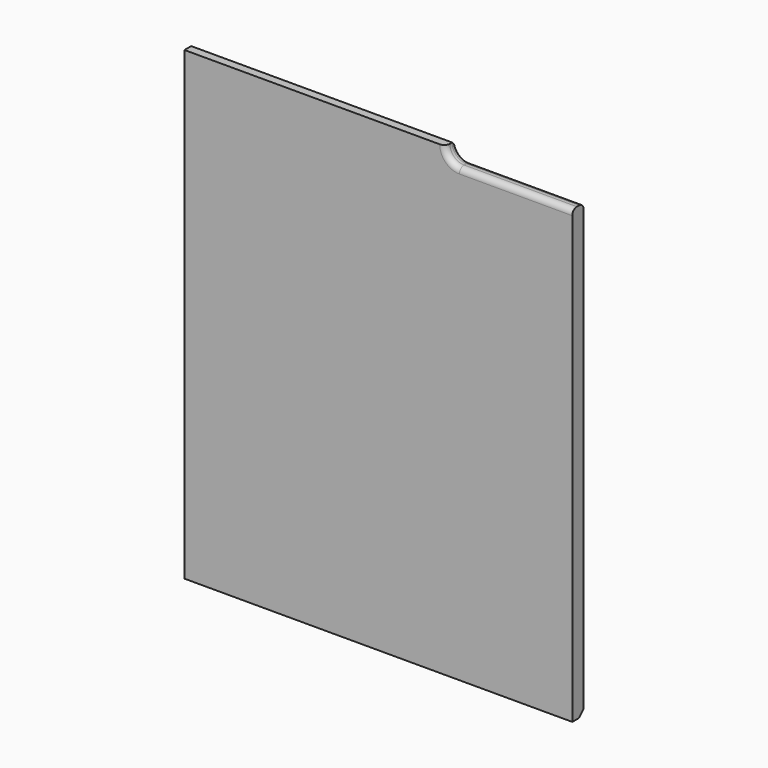
from build123d import *

# Parameters (mm, degrees)
F1_DEPTH    = 12.7
F2_R        = 5.08
F3_T1_DEPTH = 255.9982991577
F3_T3_DEPTH = 445.2282991577
F3_T5_DEPTH = 375.3782991577


# Not quite as in the source:
# - a fillet or chamfer that OpenCascade refuses, or shapes differently, is made with other operations: its cross-section is extruded or revolved along the edge and cut away or added


with BuildPart() as f1:
    # F0 (on Front) → F1 (new body)
    with BuildSketch(Plane.XZ):
        with BuildLine():
            Line((55.5559131622, 244.2450298561), (-179.3940868378, 244.2450298561))
            Line((-179.3940868378, 244.2450298561), (-179.3940868378, -174.8549701439))
            Line((-179.3940868378, -174.8549701439), (169.8559131622, -174.8549701439))
            Line((169.8559131622, -174.8549701439), (169.8559131622, 231.5450298561))
            Line((169.8559131622, 231.5450298561), (68.2559131622, 231.5450298561))
            ThreePointArc((68.2559131622, 231.5450298561), (59.2756570412, 235.264773735), (55.5559131622, 244.2450298561))
        make_face()
    extrude(amount=F1_DEPTH)

    # F2
    f2_edges = [f1.edges().sort_by_distance(p)[0] for p in [
        (119.055913, 0, 231.54503),
        (119.055913, -12.7, 231.54503),
        (59.275657, 0, 235.264774),
        (59.275657, -12.7, 235.264774),
    ]]
    fillet(f2_edges, radius=F2_R)

    # F3: chamfer of 5.08 on 3 edges, made by hand

    # F3_s2 → F3_t1 (cut)
    with BuildSketch(Plane.YZ.offset(-192.4582364166)):
        Polygon((-5.08, 244.2450298561), (0, 239.1650298561), (0, 244.2450298561), align=None)
    extrude(amount=F3_T1_DEPTH, mode=Mode.SUBTRACT)

    # F3_s4 → F3_t3 (cut)
    with BuildSketch(Plane.XY.offset(-187.9191197228)):
        Polygon((-174.3140868378, 0), (-179.3940868378, -5.08), (-179.3940868378, 0), align=None)
    extrude(amount=F3_T3_DEPTH, mode=Mode.SUBTRACT)

    # F3_s6 → F3_t5 (cut)
    with BuildSketch(Plane.YZ.offset(-192.4582364166)):
        Polygon((0, -169.7749701439), (-5.08, -174.8549701439), (0, -174.8549701439), align=None)
    extrude(amount=F3_T5_DEPTH, mode=Mode.SUBTRACT)


solid = f1.part
